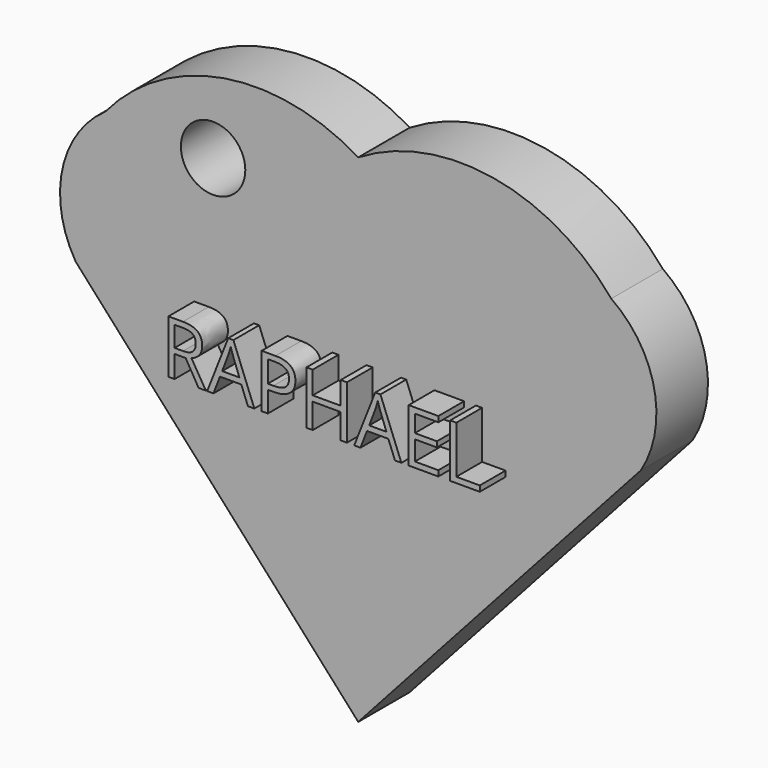
from build123d import *

# Parameters (mm, degrees)
F0_R         = 2
F1_DEPTH     = 4
F0_TEXT_SIZE = 4.6274966782
F2_DEPTH     = 6


# Not quite as in the source:
# - Text() gives the source's letters only with a copy of the font that has no kerning and outlines rounded to 1/6400 em; it was checked with that copy


with BuildPart() as f1:
    # F0 (on Front) → F1 (new body)
    with BuildSketch(Plane.XZ):
        with BuildLine():
            ThreePointArc((15.707956627, 15.8514399081), (8.3398067203, 20.0790601253), (0, 18.4635015167))
            ThreePointArc((0, 18.4635015167), (-8.3398067203, 20.0790601253), (-15.707956627, 15.8514399081))
            ThreePointArc((-15.707956627, 15.8514399081), (-18.3744318187, 11.8240667799), (-17.546365714, 7.0654818235))
            Line((-17.546365714, 7.0654818235), (0, -12.3913846154))
            Line((0, -12.3913846154), (17.546365714, 7.0654818235))
            ThreePointArc((17.546365714, 7.0654818235), (18.3744318187, 11.8240667799), (15.707956627, 15.8514399081))
        make_face()
        with BuildLine():
            Line((-9.1109837208, 5.3462386761), (-9.8007699444, 5.3462386761))
            Line((-9.8007699444, 5.3462386761), (-9.8007699444, 3.9724505997))
            Line((-9.8007699444, 3.9724505997), (-10.1847075594, 3.9724505997))
            Line((-10.1847075594, 3.9724505997), (-10.1847075594, 7.2760494001))
            Line((-10.1847075594, 7.2760494001), (-9.2787304754, 7.2760494001))
            add(Edge.make_bspline(
                [(-9.2787304754, 7.2760494001), (-8.67064849, 7.2760494001), (-8.3803453781, 7.0432284735)],
                knots=[0, 0, 0, 1, 1, 1], degree=2))
            add(Edge.make_bspline(
                [(-8.3803453781, 7.0432284735), (-8.0900422662, 6.8104075469), (-8.0900422662, 6.3425965546)],
                knots=[0, 0, 0, 1, 1, 1], degree=2))
            add(Edge.make_bspline(
                [(-8.0900422662, 6.3425965546), (-8.0900422662, 5.6875165561), (-8.7545218673, 5.4568647685)],
                knots=[0, 0, 0, 1, 1, 1], degree=2))
            Line((-8.7545218673, 5.4568647685), (-7.8572213396, 3.9724505997))
            Line((-7.8572213396, 3.9724505997), (-8.3112944511, 3.9724505997))
            Line((-8.3112944511, 3.9724505997), (-9.1109837208, 5.3462386761))
        make_face(mode=Mode.SUBTRACT)
        Polygon((-4.8500715451, 3.9724505997), (-5.2477470409, 3.9724505997), (-5.6591604174, 5.023036955), (-6.9830582952, 5.023036955), (-7.3894103472, 3.9724505997), (-7.7784092868, 3.9724505997), (-6.4725875679, 7.2897872809), (-6.1493858468, 7.2897872809), align=None, mode=Mode.SUBTRACT)
        with BuildLine():
            add(Edge.make_bspline(
                [(-3.5391885017, 7.2760494001), (-2.3013331403, 7.2760494001), (-2.3013331403, 6.3136747004)],
                knots=[0, 0, 0, 1, 1, 1], degree=2))
            add(Edge.make_bspline(
                [(-2.3013331403, 6.3136747004), (-2.3013331403, 5.8118805293), (-2.6436955899, 5.5418227154)],
                knots=[0, 0, 0, 1, 1, 1], degree=2))
            add(Edge.make_bspline(
                [(-2.6436955899, 5.5418227154), (-2.9860580394, 5.2717649014), (-3.623061879, 5.2717649014)],
                knots=[0, 0, 0, 1, 1, 1], degree=2))
            Line((-3.623061879, 5.2717649014), (-4.0120608185, 5.2717649014))
            Line((-4.0120608185, 5.2717649014), (-4.0120608185, 3.9724505997))
            Line((-4.0120608185, 3.9724505997), (-4.3959984336, 3.9724505997))
            Line((-4.3959984336, 3.9724505997), (-4.3959984336, 7.2760494001))
            Line((-4.3959984336, 7.2760494001), (-3.5391885017, 7.2760494001))
        make_face(mode=Mode.SUBTRACT)
        Polygon((0.8981469848, 7.2760494001), (0.8981469848, 3.9724505997), (0.5142093698, 3.9724505997), (0.5142093698, 5.5270002651), (-1.226163209, 5.5270002651), (-1.226163209, 3.9724505997), (-1.610100824, 3.9724505997), (-1.610100824, 7.2760494001), (-1.226163209, 7.2760494001), (-1.226163209, 5.8704472841), (0.5142093698, 5.8704472841), (0.5142093698, 7.2760494001), align=None, mode=Mode.SUBTRACT)
        with Locations((-9.0106702771, 15.4837103211)):
            Circle(F0_R, mode=Mode.SUBTRACT)
        Polygon((4.2783886989, 3.9724505997), (3.8807132032, 3.9724505997), (3.4692998266, 5.023036955), (2.1454019488, 5.023036955), (1.7390498968, 3.9724505997), (1.3500509573, 3.9724505997), (2.6558726761, 7.2897872809), (2.9790743973, 7.2897872809), align=None, mode=Mode.SUBTRACT)
        Polygon((6.5740608791, 4.3158976188), (6.5740608791, 3.9724505997), (4.7324618105, 3.9724505997), (4.7324618105, 7.2760494001), (6.5740608791, 7.2760494001), (6.5740608791, 6.9347715201), (5.1163994255, 6.9347715201), (5.1163994255, 5.8704472841), (6.4858492237, 5.8704472841), (6.4858492237, 5.5313385432), (5.1163994255, 5.5313385432), (5.1163994255, 4.3158976188), align=None, mode=Mode.SUBTRACT)
        Polygon((9.14738286, 3.9724505997), (7.3057837913, 3.9724505997), (7.3057837913, 7.2760494001), (7.6897214064, 7.2760494001), (7.6897214064, 4.320235897), (9.14738286, 4.320235897), align=None, mode=Mode.SUBTRACT)
    extrude(amount=F1_DEPTH)


with BuildPart() as f1b:
    # F0 (on Front) → F1, piece 2 (new body)
    with BuildSketch(Plane.XZ):
        with BuildLine():
            Line((-6.8471255803, 5.3686531131), (-5.7784630662, 5.3686531131))
            Line((-5.7784630662, 5.3686531131), (-6.1631237275, 6.3924867532))
            add(Edge.make_bspline(
                [(-6.1631237275, 6.3924867532), (-6.2375975022, 6.5869862229), (-6.316409555, 6.8689743017)],
                knots=[0, 0, 0, 1, 1, 1], degree=2))
            add(Edge.make_bspline(
                [(-6.316409555, 6.8689743017), (-6.3662997536, 6.6520603949), (-6.4588496871, 6.3924867532)],
                knots=[0, 0, 0, 1, 1, 1], degree=2))
            Line((-6.4588496871, 6.3924867532), (-6.8471255803, 5.3686531131))
        make_face()
    extrude(amount=F1_DEPTH)


with BuildPart() as f1c:
    # F0 (on Front) → F1, piece 3 (new body)
    with BuildSketch(Plane.XZ):
        with BuildLine():
            Line((-9.8007699444, 6.9391097983), (-9.8007699444, 5.6759478144))
            Line((-9.8007699444, 5.6759478144), (-9.2736691509, 5.6759478144))
            add(Edge.make_bspline(
                [(-9.2736691509, 5.6759478144), (-8.8673170988, 5.6759478144), (-8.6775174304, 5.837548675)],
                knots=[0, 0, 0, 1, 1, 1], degree=2))
            add(Edge.make_bspline(
                [(-8.6775174304, 5.837548675), (-8.487717762, 5.9991495355), (-8.487717762, 6.3223512566)],
                knots=[0, 0, 0, 1, 1, 1], degree=2))
            add(Edge.make_bspline(
                [(-8.487717762, 6.3223512566), (-8.487717762, 6.6498912559), (-8.680771139, 6.7945005271)],
                knots=[0, 0, 0, 1, 1, 1], degree=2))
            add(Edge.make_bspline(
                [(-8.680771139, 6.7945005271), (-8.873824516, 6.9391097983), (-9.3011449124, 6.9391097983)],
                knots=[0, 0, 0, 1, 1, 1], degree=2))
            Line((-9.3011449124, 6.9391097983), (-9.8007699444, 6.9391097983))
        make_face()
    extrude(amount=F1_DEPTH)


with BuildPart() as f1d:
    # F0 (on Front) → F1, piece 4 (new body)
    with BuildSketch(Plane.XZ):
        with BuildLine():
            Line((-4.0120608185, 6.9434480764), (-4.0120608185, 5.6014740397))
            Line((-4.0120608185, 5.6014740397), (-3.665721614, 5.6014740397))
            add(Edge.make_bspline(
                [(-3.665721614, 5.6014740397), (-3.1552508867, 5.6014740397), (-2.9271297614, 5.7663286089)],
                knots=[0, 0, 0, 1, 1, 1], degree=2))
            add(Edge.make_bspline(
                [(-2.9271297614, 5.7663286089), (-2.6990086361, 5.931183178), (-2.6990086361, 6.2955985415)],
                knots=[0, 0, 0, 1, 1, 1], degree=2))
            add(Edge.make_bspline(
                [(-2.6990086361, 6.2955985415), (-2.6990086361, 6.6231385407), (-2.9137534038, 6.7832933086)],
                knots=[0, 0, 0, 1, 1, 1], degree=2))
            add(Edge.make_bspline(
                [(-2.9137534038, 6.7832933086), (-3.1284981716, 6.9434480764), (-3.5825712831, 6.9434480764)],
                knots=[0, 0, 0, 1, 1, 1], degree=2))
            Line((-3.5825712831, 6.9434480764), (-4.0120608185, 6.9434480764))
        make_face()
    extrude(amount=F1_DEPTH)


with BuildPart() as f1e:
    # F0 (on Front) → F1, piece 5 (new body)
    with BuildSketch(Plane.XZ):
        with BuildLine():
            Line((2.2813346638, 5.3686531131), (3.3499971779, 5.3686531131))
            Line((3.3499971779, 5.3686531131), (2.9653365165, 6.3924867532))
            add(Edge.make_bspline(
                [(2.9653365165, 6.3924867532), (2.8908627418, 6.5869862229), (2.812050689, 6.8689743017)],
                knots=[0, 0, 0, 1, 1, 1], degree=2))
            add(Edge.make_bspline(
                [(2.812050689, 6.8689743017), (2.7621604905, 6.6520603949), (2.6696105569, 6.3924867532)],
                knots=[0, 0, 0, 1, 1, 1], degree=2))
            Line((2.6696105569, 6.3924867532), (2.2813346638, 5.3686531131))
        make_face()
    extrude(amount=F1_DEPTH)


with BuildPart() as f2:
    # F0 (on Front) → F2 (new body)
    with BuildSketch(Plane.XZ):
        with Locations((-10.6387806709, 3.9724505997)):
            Text('RAPHAEL', F0_TEXT_SIZE, font='Open Sans', text_align=(TextAlign.LEFT, TextAlign.BOTTOM))
    extrude(amount=F2_DEPTH)


solid = Compound([f1.part, f1b.part, f1c.part, f1d.part, f1e.part, f2.part])
